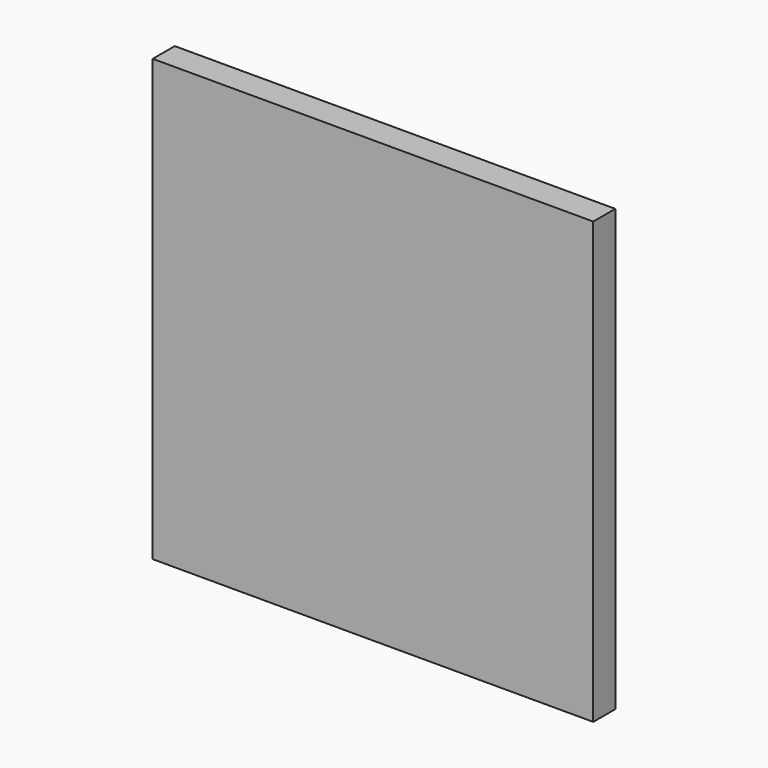
from build123d import *

# Parameters (mm, degrees)
F0_W     = 76.2
F0_H     = 76.2
F1_DEPTH = 4.7625


# Not quite as in the source:
# - a length typed as a fraction of an inch, garbled in the dataset ("3 / 203.2 mm" for 3/8 in), is restored


with BuildPart() as f1:
    # F0 (on Front) → F1 (new body)
    with BuildSketch(Plane.XZ):
        with Locations((38.1, 38.1)):
            Rectangle(F0_W, F0_H)
    extrude(amount=F1_DEPTH)


solid = f1.part
